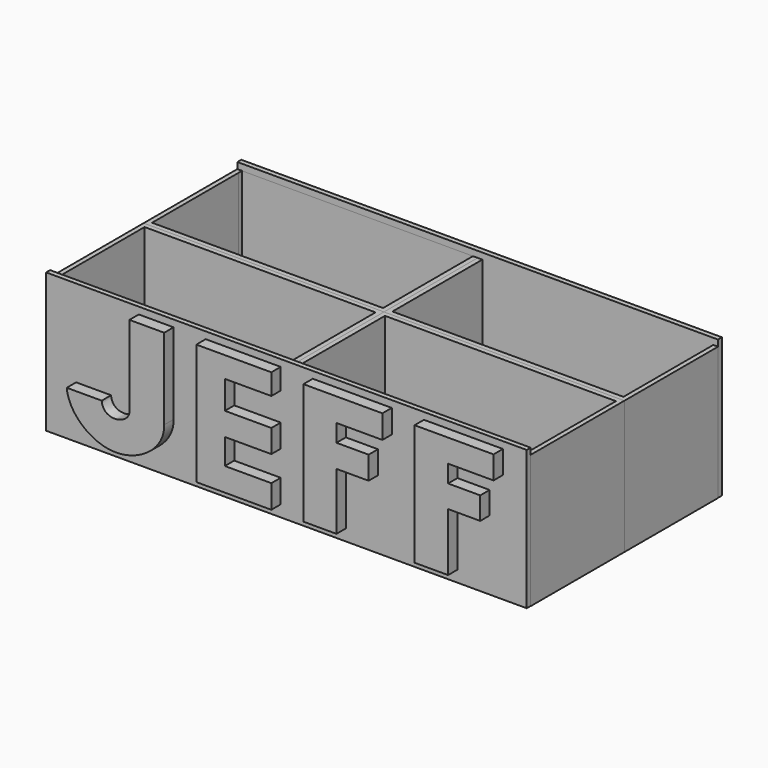
from build123d import *

# Parameters (mm, degrees)
F1_DEPTH      = 6.35
F2_W          = 2.6693828404
F2_H          = 75.5151826888
F3_DEPTH      = 152.4
F3_DEPTH_BACK = 107.95
F4_W          = 130.2241440862
F4_H          = 63.4616059251
F5_DEPTH      = 50.8
F6_DEPTH      = 21.3868
F7_T          = -2.54


# Not quite as in the source:
# - a shell that OpenCascade refuses in one call is made with other operations: the cavity is built on its own and cut out


with BuildPart() as f1:
    # F0 (on Front) → F1 (new body)
    with BuildSketch(Plane.XZ):
        with BuildLine():
            Line((-57.7272735536, 50.4536367953), (-57.7272735536, 49.0681789815))
            Line((-57.7272735536, 49.0681789815), (-57.7272735536, 6.3500003889))
            add(Edge.make_bspline(
                [(-57.7272735536, 6.3500003889), (-58.1890903413, 0), (-72.0436349511, -2.4245455861), (-72.7363601327, 7.0427274331)],
                knots=[0, 0, 0, 0, 15.0250640829, 15.0250640829, 15.0250640829, 15.0250640829], degree=3))
            Line((-72.7363601327, 7.0427274331), (-91.6709080338, 7.0427274331))
            add(Edge.make_bspline(
                [(-91.6709080338, 7.0427274331), (-90.6300544739, -4.2879367247), (-67.0665278584, -25.1007612075), (-38.6208631098, -6.0298712924), (-38.8697087765, 6.5230050582)],
                knots=[0, 0, 0, 0, 0.4971511298, 1, 1, 1, 1], degree=3))
            Line((-38.8697087765, 6.5230050582), (-38.8697087765, 50.4536367953))
            Line((-38.8697087765, 50.4536367953), (-57.7272735536, 50.4536367953))
        make_face()
    extrude(amount=F1_DEPTH)


with BuildPart() as f1b:
    # F0 (on Front) → F1, piece 2 (new body)
    with BuildSketch(Plane.XZ):
        Polygon((-21.4745458215, 50.4536367953), (-21.4745458215, -15.1245463639), (19.1654544324, -15.1245463639), (19.1654544324, -2.4245455861), (-6.0036364011, -2.4245455861), (-6.0036364011, 11.4300008863), (19.1654544324, 11.4300008863), (19.1654544324, 23.899089545), (-6.0036364011, 23.899089545), (-6.0036364011, 39.1390919685), (19.1654544324, 39.1390919685), (19.1654544324, 50.4536367953), align=None)
    extrude(amount=F1_DEPTH)


with BuildPart() as f1c:
    # F0 (on Front) → F1, piece 3 (new body)
    with BuildSketch(Plane.XZ):
        Polygon((36.5311764181, 50.4536367953), (36.5311764181, -15.1245463639), (54.4482171535, -15.1245463639), (54.4482171535, 15.868736431), (71.8675628304, 15.868736431), (71.8675628304, 28.3111259341), (54.4482171535, 28.3111259341), (54.4482171535, 37.7673432231), (79.3329998851, 37.7673432231), (79.3329998851, 50.4536367953), align=None)
    extrude(amount=F1_DEPTH)


with BuildPart() as f1d:
    # F0 (on Front) → F1, piece 4 (new body)
    with BuildSketch(Plane.XZ):
        Polygon((139.5541727543, 50.4536367953), (96.752345562, 50.4536367953), (96.752345562, -15.1245463639), (114.9182394147, -15.1245463639), (114.9182394147, 16.3664314896), (132.3375850916, 16.3664314896), (132.3375850916, 28.5599734634), (114.9182394147, 28.5599734634), (114.9182394147, 38.0161888897), (139.5541727543, 38.0161888897), align=None)
    extrude(amount=F1_DEPTH)


with BuildPart() as f3:
    # F2 (on Right) → F3 (new body, two sides)
    with BuildSketch(Plane.YZ) as f3_sk:
        with Locations((1.3346914202, 16.4288422093)):
            Rectangle(F2_W, F2_H)
    extrude(amount=F3_DEPTH)
    extrude(f3_sk.sketch, amount=-F3_DEPTH_BACK)

    # F4 (on Top) → F5 (join)
    with BuildSketch(Plane.XY):
        with Locations((-42.8596409038, 34.3579554465)):
            Rectangle(F4_W, F4_H)
    extrude(amount=F5_DEPTH)

    # F4 (on Top) → F6 (join)
    with BuildSketch(Plane.XY):
        with Locations((-42.8596409038, 34.3579554465)):
            Rectangle(F4_W, F4_H)
    extrude(amount=-F6_DEPTH)

    # F7: a shell. OpenCascade refuses it in one call, so the cavity is built on its own and cut out:
    # the body offset inwards by the wall thickness, plus a prism from it out through each open face.
    f7_core = offset(f3.part, amount=F7_T, kind=Kind.INTERSECTION, mode=Mode.PRIVATE)
    f7_exits = [f7_core.faces().sort_by_distance(p)[0] for p in [
        (-42.859173, 33.044597, 48.26),
    ]]
    add(f7_core, mode=Mode.SUBTRACT)
    extrude(f7_exits, amount=-F7_T, mode=Mode.SUBTRACT)


with BuildPart() as f8_1:
    # F8: instance of F3
    add(f3.part.mirror(Plane(origin=(22.2524311393, 34.3790536331, 14.7065806878), x_dir=(0, 1, 0), z_dir=(1, 0, 0))))


with BuildPart() as f9_1:
    # F9: instance of F8_1
    add(f8_1.part.mirror(Plane(origin=(87.3645031825, 66.088758409, 14.7066), x_dir=(-1, 0, 0), z_dir=(0, 1, 0))))


with BuildPart() as f9_2:
    # F9: instance of F3
    add(f3.part.mirror(Plane(origin=(87.3645031825, 66.088758409, 14.7066), x_dir=(-1, 0, 0), z_dir=(0, 1, 0))))


solid = Compound([f1.part, f1b.part, f1c.part, f1d.part, f3.part, f8_1.part, f9_1.part, f9_2.part])
